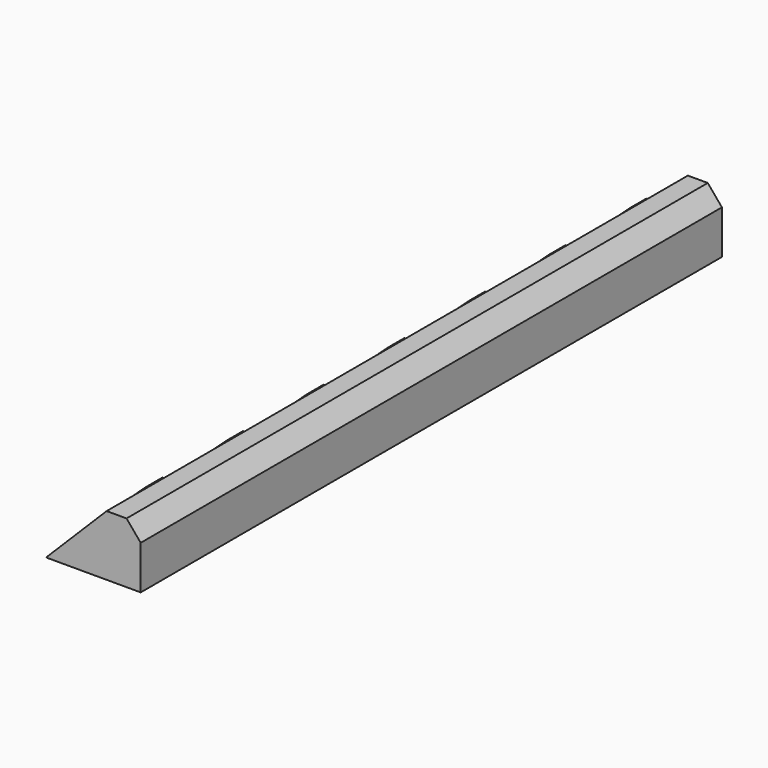
from build123d import *

# Parameters (mm, degrees)
F1_DEPTH = 457.2
F2_W     = 5.08
F2_H     = 19.05
F3_DEPTH = 3.175


# Not quite as in the source:
# - a length typed as a fraction of an inch, garbled in the dataset ("3 / 203.2 mm" for 3/8 in), is restored


with BuildPart() as f1:
    # F0 (on Front) → F1 (new body, symmetric)
    with BuildSketch(Plane.XZ):
        Polygon((-76.2, 0), (0, 0), (42.8860933474, 0), (42.8860933474, 54.9768594564), (25.0777639449, 76.2), (0, 76.2), align=None)
    extrude(amount=F1_DEPTH, both=True)

    # F2 (on face) → F3 (join)
    with BuildSketch(Plane(origin=(-38.1, 0, 38.1), x_dir=(0, -1, 0), z_dir=(-0.7071067812, 0, 0.7071067812))):
        with BuildLine():
            Line((-391.6987875515, 28.4815367264), (-417.0987875515, 28.4815367264))
            ThreePointArc((-417.0987875515, 28.4815367264), (-431.8, -3.2684632736), (-417.0987875515, -35.0184632736))
            Line((-417.0987875515, -35.0184632736), (-391.6987875515, -35.0184632736))
            ThreePointArc((-391.6987875515, -35.0184632736), (-376.9975751031, -3.2684632736), (-391.6987875515, 28.4815367264))
        make_face()
        with BuildLine():
            Line((-400.5195509719, -30.7538155466), (-409.9965240192, -30.7538155466))
            Line((-409.9965240192, -30.7538155466), (-409.9965240192, -25.4346902415))
            ThreePointArc((-409.9965240192, -25.4346902415), (-405.2253041336, -20.6960921992), (-400.5195509719, -25.4997093556))
            Line((-400.5195509719, -25.4997093556), (-400.5195509719, -30.7538155466))
        make_face(mode=Mode.SUBTRACT)
        with Locations((-412.5365240192, 2.0394300796)):
            Rectangle(F2_W, F2_H, mode=Mode.SUBTRACT)
        with Locations((-397.9795509719, 2.4147130909)):
            Rectangle(F2_W, F2_H, mode=Mode.SUBTRACT)
        with BuildLine():
            Line((-264.41702, 28.96613), (-289.81702, 28.96613))
            ThreePointArc((-289.81702, 28.96613), (-304.5182324485, -2.78387), (-289.81702, -34.53387))
            Line((-289.81702, -34.53387), (-264.41702, -34.53387))
            ThreePointArc((-264.41702, -34.53387), (-249.7158075515, -2.78387), (-264.41702, 28.96613))
        make_face()
        with BuildLine():
            Line((-272.8882718836, -29.7792267651), (-282.365244931, -29.7792267651))
            Line((-282.365244931, -29.7792267651), (-282.365244931, -24.46010146))
            ThreePointArc((-282.365244931, -24.46010146), (-277.5940250453, -19.7215034177), (-272.8882718836, -24.5251205741))
            Line((-272.8882718836, -24.5251205741), (-272.8882718836, -29.7792267651))
        make_face(mode=Mode.SUBTRACT)
        with Locations((-284.905244931, 3.0140188611)):
            Rectangle(F2_W, F2_H, mode=Mode.SUBTRACT)
        with Locations((-270.3482718836, 3.3893018724)):
            Rectangle(F2_W, F2_H, mode=Mode.SUBTRACT)
        with BuildLine():
            Line((-137.1352524485, 29.4507232736), (-162.5352524485, 29.4507232736))
            ThreePointArc((-162.5352524485, 29.4507232736), (-177.2364648969, -2.2992767264), (-162.5352524485, -34.0492767264))
            Line((-162.5352524485, -34.0492767264), (-137.1352524485, -34.0492767264))
            ThreePointArc((-137.1352524485, -34.0492767264), (-122.43404, -2.2992767264), (-137.1352524485, 29.4507232736))
        make_face()
        with BuildLine():
            Line((-145.2569927954, -28.8046379836), (-154.7339658427, -28.8046379836))
            Line((-154.7339658427, -28.8046379836), (-154.7339658427, -23.4855126785))
            ThreePointArc((-154.7339658427, -23.4855126785), (-149.962745957, -18.7469146362), (-145.2569927954, -23.5505317926))
            Line((-145.2569927954, -23.5505317926), (-145.2569927954, -28.8046379836))
        make_face(mode=Mode.SUBTRACT)
        with Locations((-157.2739658427, 3.9886076427)):
            Rectangle(F2_W, F2_H, mode=Mode.SUBTRACT)
        with Locations((-142.7169927954, 4.3638906539)):
            Rectangle(F2_W, F2_H, mode=Mode.SUBTRACT)
        with BuildLine():
            Line((-9.8534848969, 29.9353165472), (-35.2534848969, 29.9353165472))
            ThreePointArc((-35.2534848969, 29.9353165472), (-49.9546973454, -1.8146834528), (-35.2534848969, -33.5646834528))
            Line((-35.2534848969, -33.5646834528), (-9.8534848969, -33.5646834528))
            ThreePointArc((-9.8534848969, -33.5646834528), (4.8477275515, -1.8146834528), (-9.8534848969, 29.9353165472))
        make_face()
        with BuildLine():
            Line((-17.6257137071, -27.8300492021), (-27.1026867544, -27.8300492021))
            Line((-27.1026867544, -27.8300492021), (-27.1026867544, -22.5109238969))
            ThreePointArc((-27.1026867544, -22.5109238969), (-22.3314668688, -17.7723258546), (-17.6257137071, -22.575943011))
            Line((-17.6257137071, -22.575943011), (-17.6257137071, -27.8300492021))
        make_face(mode=Mode.SUBTRACT)
        with Locations((-29.6426867544, 4.9631964242)):
            Rectangle(F2_W, F2_H, mode=Mode.SUBTRACT)
        with Locations((-15.0857137071, 5.3384794355)):
            Rectangle(F2_W, F2_H, mode=Mode.SUBTRACT)
        with BuildLine():
            Line((117.4282826546, 30.4199098208), (92.0282826546, 30.4199098208))
            ThreePointArc((92.0282826546, 30.4199098208), (77.3270702061, -1.3300901792), (92.0282826546, -33.0800901792))
            Line((92.0282826546, -33.0800901792), (117.4282826546, -33.0800901792))
            ThreePointArc((117.4282826546, -33.0800901792), (132.1294951031, -1.3300901792), (117.4282826546, 30.4199098208))
        make_face()
        with BuildLine():
            Line((110.0055653812, -26.8554604205), (100.5285923338, -26.8554604205))
            Line((100.5285923338, -26.8554604205), (100.5285923338, -21.5363351154))
            ThreePointArc((100.5285923338, -21.5363351154), (105.2998122195, -16.7977370731), (110.0055653812, -21.6013542295))
            Line((110.0055653812, -21.6013542295), (110.0055653812, -26.8554604205))
        make_face(mode=Mode.SUBTRACT)
        with Locations((97.9885923338, 5.9377852057)):
            Rectangle(F2_W, F2_H, mode=Mode.SUBTRACT)
        with Locations((112.5455653812, 6.313068217)):
            Rectangle(F2_W, F2_H, mode=Mode.SUBTRACT)
        with BuildLine():
            Line((244.7100502061, 30.9045030943), (219.3100502061, 30.9045030943))
            ThreePointArc((219.3100502061, 30.9045030943), (204.6088377576, -0.8454969057), (219.3100502061, -32.5954969057))
            Line((219.3100502061, -32.5954969057), (244.7100502061, -32.5954969057))
            ThreePointArc((244.7100502061, -32.5954969057), (259.4112626546, -0.8454969057), (244.7100502061, 30.9045030943))
        make_face()
        with BuildLine():
            Line((237.6368444694, -25.880871639), (228.1598714221, -25.880871639))
            Line((228.1598714221, -25.880871639), (228.1598714221, -20.5617463339))
            ThreePointArc((228.1598714221, -20.5617463339), (232.9310913078, -15.8231482916), (237.6368444694, -20.626765448))
            Line((237.6368444694, -20.626765448), (237.6368444694, -25.880871639))
        make_face(mode=Mode.SUBTRACT)
        with Locations((225.6198714221, 6.9123739872)):
            Rectangle(F2_W, F2_H, mode=Mode.SUBTRACT)
        with Locations((240.1768444694, 7.2876569985)):
            Rectangle(F2_W, F2_H, mode=Mode.SUBTRACT)
        with BuildLine():
            Line((371.9918177576, 31.3890963679), (346.5918177576, 31.3890963679))
            ThreePointArc((346.5918177576, 31.3890963679), (331.8906053092, -0.3609036321), (346.5918177576, -32.1109036321))
            Line((346.5918177576, -32.1109036321), (371.9918177576, -32.1109036321))
            ThreePointArc((371.9918177576, -32.1109036321), (386.6930302061, -0.3609036321), (371.9918177576, 31.3890963679))
        make_face()
        with BuildLine():
            Line((365.2681235577, -24.9062828575), (355.7911505104, -24.9062828575))
            Line((355.7911505104, -24.9062828575), (355.7911505104, -19.5871575524))
            ThreePointArc((355.7911505104, -19.5871575524), (360.562370396, -14.8485595101), (365.2681235577, -19.6521766665))
            Line((365.2681235577, -19.6521766665), (365.2681235577, -24.9062828575))
        make_face(mode=Mode.SUBTRACT)
        with Locations((353.2511505104, 7.8869627688)):
            Rectangle(F2_W, F2_H, mode=Mode.SUBTRACT)
        with Locations((367.8081235577, 8.26224578)):
            Rectangle(F2_W, F2_H, mode=Mode.SUBTRACT)
    extrude(amount=F3_DEPTH)


solid = f1.part
